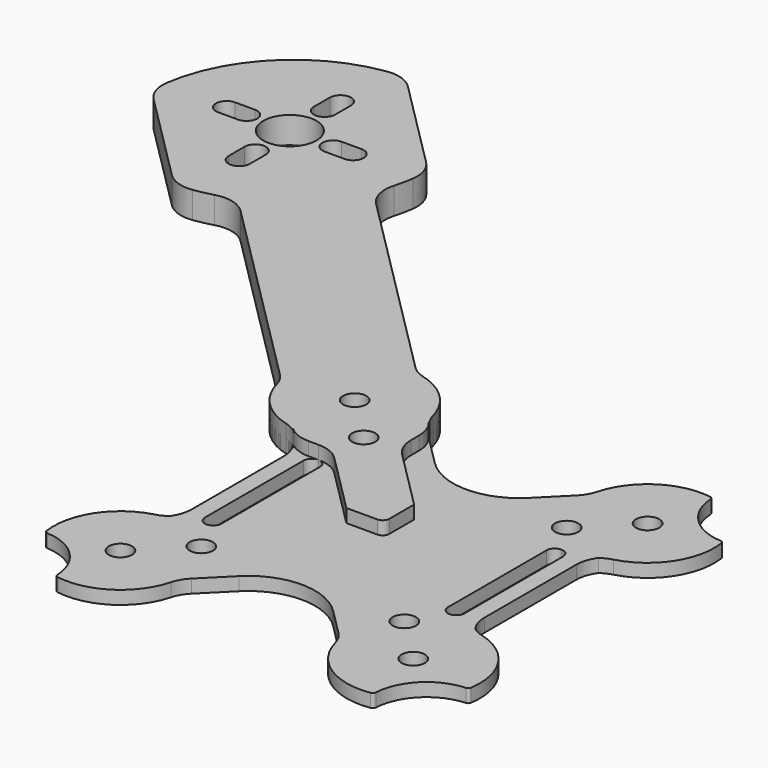
from build123d import *

# Parameters (mm, degrees)
F0_R     = 1.75
F0_R_2   = 4
F1_DEPTH = 4
F2_R     = 5
F3_R     = 1
F4_R     = 1.75
F5_DEPTH = 2


with BuildPart() as f1:
    # F0 (on Top) → F1 (new body)
    with BuildSketch(Plane.XY):
        with BuildLine():
            Line((-21.6346483726, 32.9483568716), (-53.4040320636, 64.7177405626))
            ThreePointArc((-53.4040320636, 64.7177405626), (-52.1203664971, 68.6888343282), (-51.6187950266, 72.8319984622))
            Line((-51.6187950266, 72.8319984622), (-68.5893577751, 89.8025612107))
            ThreePointArc((-68.5893577751, 89.8025612107), (-83.43860018, 83.43860018), (-89.8025612107, 68.5893577751))
            Line((-89.8025612107, 68.5893577751), (-72.8319984622, 51.6187950266))
            ThreePointArc((-72.8319984622, 51.6187950266), (-68.6888343282, 52.1203664971), (-64.7177405626, 53.4040320636))
            Line((-64.7177405626, 53.4040320636), (-32.9483568716, 21.6346483726))
            ThreePointArc((-32.9483568716, 21.6346483726), (-32.1553695931, 20.6018937928), (-31.655927185, 19.3994096445))
            ThreePointArc((-31.655927185, 19.3994096445), (-29.0710678119, 14.9289321881), (-24.6005903555, 12.344072815))
            ThreePointArc((-24.6005903555, 12.344072815), (-23.3981062072, 11.8446304069), (-22.3653516274, 11.0516431284))
            Line((-22.3653516274, 11.0516431284), (-23.2781745931, 11.9644660941))
            ThreePointArc((-23.2781745931, 11.9644660941), (-21.6560578489, 10.8806023374), (-19.7426406871, 10.5))
            Line((-19.7426406871, 10.5), (-18.2279220614, 10.5))
            ThreePointArc((-18.2279220614, 10.5), (-16.3145048995, 10.1193976626), (-14.6923881554, 9.0355339059))
            Line((-14.6923881554, 9.0355339059), (-5.6568542495, 0))
            Line((-5.6568542495, 0), (0, 0))
            Line((0, 0), (0, 5.6568542495))
            Line((0, 5.6568542495), (-9.0355339059, 14.6923881554))
            ThreePointArc((-9.0355339059, 14.6923881554), (-10.1193976626, 16.3145048995), (-10.5, 18.2279220614))
            Line((-10.5, 18.2279220614), (-10.5, 19.7426406871))
            ThreePointArc((-10.5, 19.7426406871), (-10.8806023374, 21.6560578489), (-11.9644660941, 23.2781745931))
            Line((-11.9644660941, 23.2781745931), (-11.0516431284, 22.3653516274))
            ThreePointArc((-11.0516431284, 22.3653516274), (-11.8446304069, 23.3981062072), (-12.344072815, 24.6005903555))
            ThreePointArc((-12.344072815, 24.6005903555), (-14.9289321881, 29.0710678119), (-19.3994096445, 31.655927185))
            ThreePointArc((-19.3994096445, 31.655927185), (-20.6018937928, 32.1553695931), (-21.6346483726, 32.9483568716))
        make_face()
        with Locations((-15.25, 15.25)):
            Circle(F0_R, mode=Mode.SUBTRACT)
        with Locations((-22, 22)):
            Circle(F0_R, mode=Mode.SUBTRACT)
        with BuildLine():
            Line((-69.1106781187, 64.2106781187), (-69.1106781187, 61.2106781187))
            ThreePointArc((-69.1106781187, 61.2106781187), (-70.7106781187, 59.6106781187), (-72.3106781187, 61.2106781187))
            Line((-72.3106781187, 61.2106781187), (-72.3106781187, 64.2106781187))
            ThreePointArc((-72.3106781187, 64.2106781187), (-70.7106781187, 65.8106781187), (-69.1106781187, 64.2106781187))
        make_face(mode=Mode.SUBTRACT)
        with BuildLine():
            Line((-77.2106781187, 69.1106781187), (-80.2106781187, 69.1106781187))
            ThreePointArc((-80.2106781187, 69.1106781187), (-81.8106781187, 70.7106781187), (-80.2106781187, 72.3106781187))
            Line((-80.2106781187, 72.3106781187), (-77.2106781187, 72.3106781187))
            ThreePointArc((-77.2106781187, 72.3106781187), (-75.6106781187, 70.7106781187), (-77.2106781187, 69.1106781187))
        make_face(mode=Mode.SUBTRACT)
        with Locations((-70.7106781187, 70.7106781187)):
            Circle(F0_R_2, mode=Mode.SUBTRACT)
        with BuildLine():
            Line((-69.1106781187, 80.2106781187), (-69.1106781187, 77.2106781187))
            ThreePointArc((-69.1106781187, 77.2106781187), (-70.7106781187, 75.6106781187), (-72.3106781187, 77.2106781187))
            Line((-72.3106781187, 77.2106781187), (-72.3106781187, 80.2106781187))
            ThreePointArc((-72.3106781187, 80.2106781187), (-70.7106781187, 81.8106781187), (-69.1106781187, 80.2106781187))
        make_face(mode=Mode.SUBTRACT)
        with BuildLine():
            Line((-64.2106781187, 72.3106781187), (-61.2106781187, 72.3106781187))
            ThreePointArc((-61.2106781187, 72.3106781187), (-59.6106781187, 70.7106781187), (-61.2106781187, 69.1106781187))
            Line((-61.2106781187, 69.1106781187), (-64.2106781187, 69.1106781187))
            ThreePointArc((-64.2106781187, 69.1106781187), (-65.8106781187, 70.7106781187), (-64.2106781187, 72.3106781187))
        make_face(mode=Mode.SUBTRACT)
    extrude(amount=F1_DEPTH)

    # F2
    f2_edges = [f1.edges().sort_by_distance(p)[0] for p in [
        (-64.717741, 53.404032, 2),
        (-53.404032, 64.717741, 2),
        (-72.831998, 51.618795, 2),
        (-51.618795, 72.831998, 2),
        (-89.802561, 68.589358, 2),
        (-68.589358, 89.802561, 2),
    ]]
    fillet(f2_edges, radius=F2_R)

    # F3
    f3_edges = [f1.edges().sort_by_distance(p)[0] for p in [
        (0, 0, 2),
    ]]
    fillet(f3_edges, radius=F3_R)


with BuildPart() as f5:
    # F4 (on Top) → F5 (new body)
    with BuildSketch(Plane.XY):
        with BuildLine():
            ThreePointArc((-11.0516431284, 22.3653516274), (-11.8446304069, 23.3981062072), (-12.344072815, 24.6005903555))
            ThreePointArc((-12.344072815, 24.6005903555), (-16.5270441555, 30.3693939042), (-23.4889823618, 31.8885252453))
            ThreePointArc((-23.4889823618, 31.8885252453), (-23.7836266036, 31.7313972067), (-23.9136486374, 31.4238281567))
            ThreePointArc((-23.9136486374, 31.4238281567), (-26.2426406871, 26.2426406871), (-31.4238281567, 23.9136486374))
            ThreePointArc((-31.4238281567, 23.9136486374), (-31.7313972067, 23.7836266036), (-31.8885252453, 23.4889823618))
            ThreePointArc((-31.8885252453, 23.4889823618), (-30.3693939042, 16.5270441555), (-24.6005903555, 12.344072815))
            ThreePointArc((-24.6005903555, 12.344072815), (-23.7431585277, 12.0265653157), (-22.9578811212, 11.5582281012))
            ThreePointArc((-22.9578811212, 11.5582281012), (-22.2454971662, 10.1627064202), (-22, 8.6152236891))
            Line((-22, 8.6152236891), (-22, 0))
            Line((-22, 0), (-22, -8.6152236891))
            ThreePointArc((-22, -8.6152236891), (-22.2454971662, -10.1627064202), (-22.9578811212, -11.5582281012))
            ThreePointArc((-22.9578811212, -11.5582281012), (-23.7431585277, -12.0265653157), (-24.6005903555, -12.344072815))
            ThreePointArc((-24.6005903555, -12.344072815), (-30.3693939042, -16.5270441555), (-31.8885252453, -23.4889823618))
            ThreePointArc((-31.8885252453, -23.4889823618), (-31.7313972067, -23.7836266036), (-31.4238281567, -23.9136486374))
            ThreePointArc((-31.4238281567, -23.9136486374), (-26.2426406871, -26.2426406871), (-23.9136486374, -31.4238281567))
            ThreePointArc((-23.9136486374, -31.4238281567), (-23.7836266036, -31.7313972067), (-23.4889823618, -31.8885252453))
            ThreePointArc((-23.4889823618, -31.8885252453), (-16.5270441555, -30.3693939042), (-12.344072815, -24.6005903555))
            ThreePointArc((-12.344072815, -24.6005903555), (-11.8446304069, -23.3981062072), (-11.0516431284, -22.3653516274))
            Line((-11.0516431284, -22.3653516274), (-7.0710678119, -18.3847763109))
            ThreePointArc((-7.0710678119, -18.3847763109), (0, -15.4558441227), (7.0710678119, -18.3847763109))
            Line((7.0710678119, -18.3847763109), (11.0516431284, -22.3653516274))
            ThreePointArc((11.0516431284, -22.3653516274), (11.8446304069, -23.3981062072), (12.344072815, -24.6005903555))
            ThreePointArc((12.344072815, -24.6005903555), (16.5270441555, -30.3693939042), (23.4889823618, -31.8885252453))
            ThreePointArc((23.4889823618, -31.8885252453), (23.7836266036, -31.7313972067), (23.9136486374, -31.4238281567))
            ThreePointArc((23.9136486374, -31.4238281567), (26.2426406871, -26.2426406871), (31.4238281567, -23.9136486374))
            ThreePointArc((31.4238281567, -23.9136486374), (31.7313972067, -23.7836266036), (31.8885252453, -23.4889823618))
            ThreePointArc((31.8885252453, -23.4889823618), (30.3693939042, -16.5270441555), (24.6005903555, -12.344072815))
            ThreePointArc((24.6005903555, -12.344072815), (23.7431585277, -12.0265653157), (22.9578811212, -11.5582281012))
            ThreePointArc((22.9578811212, -11.5582281012), (22.2454971662, -10.1627064202), (22, -8.6152236891))
            Line((22, -8.6152236891), (22, 0))
            Line((22, 0), (22, 8.6152236891))
            ThreePointArc((22, 8.6152236891), (22.2454971662, 10.1627064202), (22.9578811212, 11.5582281012))
            ThreePointArc((22.9578811212, 11.5582281012), (23.7431585277, 12.0265653157), (24.6005903555, 12.344072815))
            ThreePointArc((24.6005903555, 12.344072815), (30.3693939042, 16.5270441555), (31.8885252453, 23.4889823618))
            ThreePointArc((31.8885252453, 23.4889823618), (31.7313972067, 23.7836266036), (31.4238281567, 23.9136486374))
            ThreePointArc((31.4238281567, 23.9136486374), (26.2426406871, 26.2426406871), (23.9136486374, 31.4238281567))
            ThreePointArc((23.9136486374, 31.4238281567), (23.7836266036, 31.7313972067), (23.4889823618, 31.8885252453))
            ThreePointArc((23.4889823618, 31.8885252453), (16.5270441555, 30.3693939042), (12.344072815, 24.6005903555))
            ThreePointArc((12.344072815, 24.6005903555), (11.8446304069, 23.3981062072), (11.0516431284, 22.3653516274))
            Line((11.0516431284, 22.3653516274), (7.0710678119, 18.3847763109))
            ThreePointArc((7.0710678119, 18.3847763109), (0, 15.4558441227), (-7.0710678119, 18.3847763109))
            Line((-7.0710678119, 18.3847763109), (-11.0516431284, 22.3653516274))
        make_face()
        with Locations((-22, -22)):
            Circle(F4_R, mode=Mode.SUBTRACT)
        with BuildLine():
            ThreePointArc((-23.4644660941, -12.1507575951), (-23.1996081476, -11.864380775), (-22.9578811212, -11.5582281012))
            ThreePointArc((-22.9578811212, -11.5582281012), (-22.6517284475, -11.3165010748), (-22.3653516274, -11.0516431284))
            Line((-22.3653516274, -11.0516431284), (-23.4644660941, -12.1507575951))
        make_face(mode=Mode.SUBTRACT)
        with Locations((-15.25, -15.25)):
            Circle(F4_R, mode=Mode.SUBTRACT)
        with Locations((22, -22)):
            Circle(F4_R, mode=Mode.SUBTRACT)
        with Locations((15.25, -15.25)):
            Circle(F4_R, mode=Mode.SUBTRACT)
        with BuildLine():
            ThreePointArc((22.3653516274, -11.0516431284), (22.6517284475, -11.3165010748), (22.9578811212, -11.5582281012))
            ThreePointArc((22.9578811212, -11.5582281012), (23.1996081476, -11.864380775), (23.4644660941, -12.1507575951))
            Line((23.4644660941, -12.1507575951), (22.3653516274, -11.0516431284))
        make_face(mode=Mode.SUBTRACT)
        with BuildLine():
            Line((-19.5, 0), (-19.5, 9.25))
            ThreePointArc((-19.5, 9.25), (-19.1338834765, 10.1338834765), (-18.25, 10.5))
            ThreePointArc((-18.25, 10.5), (-17.3661165235, 10.1338834765), (-17, 9.25))
            Line((-17, 9.25), (-17, 0))
            Line((-17, 0), (-17, -9.25))
            ThreePointArc((-17, -9.25), (-17.3661165235, -10.1338834765), (-18.25, -10.5))
            ThreePointArc((-18.25, -10.5), (-19.1338834765, -10.1338834765), (-19.5, -9.25))
            Line((-19.5, -9.25), (-19.5, 0))
        make_face(mode=Mode.SUBTRACT)
        with BuildLine():
            ThreePointArc((-22.3653516274, 11.0516431284), (-22.6517284475, 11.3165010748), (-22.9578811212, 11.5582281012))
            ThreePointArc((-22.9578811212, 11.5582281012), (-23.1996081476, 11.864380775), (-23.4644660941, 12.1507575951))
            Line((-23.4644660941, 12.1507575951), (-22.3653516274, 11.0516431284))
        make_face(mode=Mode.SUBTRACT)
        with Locations((-15.25, 15.25)):
            Circle(F4_R, mode=Mode.SUBTRACT)
        with Locations((-22, 22)):
            Circle(F4_R, mode=Mode.SUBTRACT)
        with Locations((15.25, 15.25)):
            Circle(F4_R, mode=Mode.SUBTRACT)
        with BuildLine():
            ThreePointArc((17, 9.25), (17.3661165235, 10.1338834765), (18.25, 10.5))
            ThreePointArc((18.25, 10.5), (19.1338834765, 10.1338834765), (19.5, 9.25))
            Line((19.5, 9.25), (19.5, 0))
            Line((19.5, 0), (19.5, -9.25))
            ThreePointArc((19.5, -9.25), (19.1338834765, -10.1338834765), (18.25, -10.5))
            ThreePointArc((18.25, -10.5), (17.3661165235, -10.1338834765), (17, -9.25))
            Line((17, -9.25), (17, 0))
            Line((17, 0), (17, 9.25))
        make_face(mode=Mode.SUBTRACT)
        with BuildLine():
            ThreePointArc((23.4644660941, 12.1507575951), (23.1996081476, 11.864380775), (22.9578811212, 11.5582281012))
            ThreePointArc((22.9578811212, 11.5582281012), (22.6517284475, 11.3165010748), (22.3653516274, 11.0516431284))
            Line((22.3653516274, 11.0516431284), (23.4644660941, 12.1507575951))
        make_face(mode=Mode.SUBTRACT)
        with Locations((22, 22)):
            Circle(F4_R, mode=Mode.SUBTRACT)
        with BuildLine():
            ThreePointArc((-23.4644660941, 12.1507575951), (-23.1996081476, 11.864380775), (-22.9578811212, 11.5582281012))
            ThreePointArc((-22.9578811212, 11.5582281012), (-22.6517284475, 11.3165010748), (-22.3653516274, 11.0516431284))
            Line((-22.3653516274, 11.0516431284), (-23.4644660941, 12.1507575951))
        make_face()
        with BuildLine():
            ThreePointArc((-22.3653516274, -11.0516431284), (-22.6517284475, -11.3165010748), (-22.9578811212, -11.5582281012))
            ThreePointArc((-22.9578811212, -11.5582281012), (-23.1996081476, -11.864380775), (-23.4644660941, -12.1507575951))
            Line((-23.4644660941, -12.1507575951), (-22.3653516274, -11.0516431284))
        make_face()
        with BuildLine():
            ThreePointArc((23.4644660941, -12.1507575951), (23.1996081476, -11.864380775), (22.9578811212, -11.5582281012))
            ThreePointArc((22.9578811212, -11.5582281012), (22.6517284475, -11.3165010748), (22.3653516274, -11.0516431284))
            Line((22.3653516274, -11.0516431284), (23.4644660941, -12.1507575951))
        make_face()
        with BuildLine():
            ThreePointArc((22.3653516274, 11.0516431284), (22.6517284475, 11.3165010748), (22.9578811212, 11.5582281012))
            ThreePointArc((22.9578811212, 11.5582281012), (23.1996081476, 11.864380775), (23.4644660941, 12.1507575951))
            Line((23.4644660941, 12.1507575951), (22.3653516274, 11.0516431284))
        make_face()
    extrude(amount=F5_DEPTH)


solid = Compound([f1.part, f5.part])
